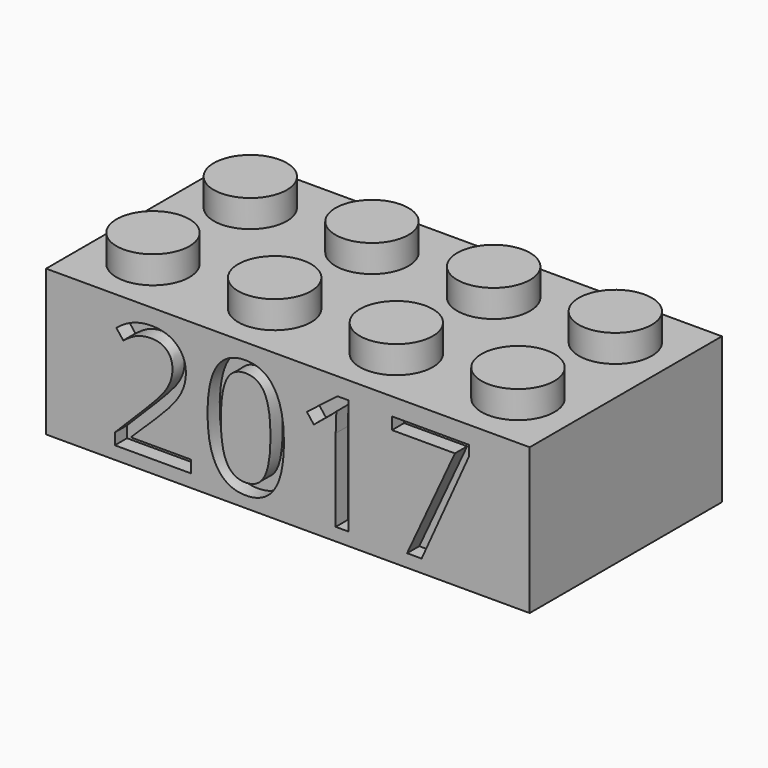
from build123d import *

# Parameters (mm, degrees)
F0_W          = 31.8
F0_H          = 15.8
F1_DEPTH      = 9.6
F2_W          = 29.4
F2_H          = 13.4
F3_DEPTH      = 8.4
F4_R          = 2.4
F5_DEPTH      = 1.8
F6_W          = 29.4
F6_H          = 13.4
F6_R          = 1.3
F7_DEPTH      = 1
F8_R          = 3.255
F9_DEPTH      = 7.4
F10_R         = 2.4
F11_DEPTH     = 7.4
F12_W         = 0.8
F12_H         = 13.4
F13_DEPTH     = 6.4
F15_DEPTH     = 6.4
F16_W         = 0.6
F16_H         = 0.3
F17_DEPTH     = 7.4
F18_W         = 0.3
F18_H         = 0.6
F19_DEPTH     = 7.4
F20_TEXT_SIZE = 9.802063729
F21_DEPTH     = 1
F22_TEXT_SIZE = 10.6435608972
F23_DEPTH     = 1


# Not quite as in the source:
# - Text() gives the source's letters only with a copy of the font that has no kerning and outlines rounded to 1/6400 em; it was checked with that copy


with BuildPart() as f1:
    # F0 (on Top) → F1 (new body)
    with BuildSketch(Plane.XY):
        Rectangle(F0_W, F0_H)
    extrude(amount=F1_DEPTH)

    # F2 (on Top) → F3 (cut)
    with BuildSketch(Plane.XY):
        Rectangle(F2_W, F2_H)
    extrude(amount=F3_DEPTH, mode=Mode.SUBTRACT)

    # F4 (on face) → F5 (join)
    with BuildSketch(Plane.XY.offset(9.6)):
        with Locations((-11.95, 3.95)):
            Circle(F4_R)
        with Locations((-11.95, -4.05)):
            Circle(F4_R)
        with Locations((-3.95, -4.05)):
            Circle(F4_R)
        with Locations((4.05, 3.95)):
            Circle(F4_R)
        with Locations((-3.95, 3.95)):
            Circle(F4_R)
        with Locations((4.05, -4.05)):
            Circle(F4_R)
        with Locations((12.05, -4.05)):
            Circle(F4_R)
        with Locations((12.05, 3.95)):
            Circle(F4_R)
    extrude(amount=F5_DEPTH)

    # F6 (on face) → F7 (join)
    with BuildSketch(Plane(origin=(0, 0, 8.4), x_dir=(1, 0, 0), z_dir=(0, 0, -1))):
        Rectangle(F6_W, F6_H)
        with Locations((-11.95, -4.05)):
            Circle(F6_R, mode=Mode.SUBTRACT)
        with Locations((-3.95, -4.05)):
            Circle(F6_R, mode=Mode.SUBTRACT)
        with Locations((4.05, -4.05)):
            Circle(F6_R, mode=Mode.SUBTRACT)
        with Locations((12.05, -4.05)):
            Circle(F6_R, mode=Mode.SUBTRACT)
        with Locations((-11.95, 3.95)):
            Circle(F6_R, mode=Mode.SUBTRACT)
        with Locations((-3.95, 3.95)):
            Circle(F6_R, mode=Mode.SUBTRACT)
        with Locations((4.05, 3.95)):
            Circle(F6_R, mode=Mode.SUBTRACT)
        with Locations((12.05, 3.95)):
            Circle(F6_R, mode=Mode.SUBTRACT)
    extrude(amount=F7_DEPTH)

    # F8 (on face) → F9 (join)
    with BuildSketch(Plane(origin=(0, 0, 7.4), x_dir=(1, 0, 0), z_dir=(0, 0, -1))):
        with Locations((7.945, 0)):
            Circle(F8_R)
        with Locations((-0.055, 0)):
            Circle(F8_R)
        with Locations((-8.055, 0)):
            Circle(F8_R)
    extrude(amount=F9_DEPTH)

    # F10 (on face) → F11 (cut)
    with BuildSketch(Plane(origin=(0, 0, 0), x_dir=(1, 0, 0), z_dir=(0, 0, -1))):
        with Locations((-8.055, 0)):
            Circle(F10_R)
        with Locations((-0.055, 0)):
            Circle(F10_R)
        with Locations((7.945, 0)):
            Circle(F10_R)
    extrude(amount=-F11_DEPTH, mode=Mode.SUBTRACT)

    # F12 (on face) → F13 (join)
    with BuildSketch(Plane(origin=(0, 0, 7.4), x_dir=(1, 0, 0), z_dir=(0, 0, -1))):
        Rectangle(F12_W, F12_H)
    extrude(amount=F13_DEPTH)

    # F14 (on face) → F15 (cut)
    with BuildSketch(Plane(origin=(0, 0, 1), x_dir=(1, 0, 0), z_dir=(0, 0, -1))):
        with BuildLine():
            Line((-0.4, 2.3750736831), (-0.4, -2.3750736831))
            ThreePointArc((-0.4, -2.3750736831), (0.0007806115, -2.3993516881), (0.4, -2.3564751219))
            Line((0.4, -2.3564751219), (0.4, 2.3564751219))
            ThreePointArc((0.4, 2.3564751219), (0.0007806115, 2.3993516881), (-0.4, 2.3750736831))
        make_face()
    extrude(amount=-F15_DEPTH, mode=Mode.SUBTRACT)

    # F16 (on face) → F17 (join, through all)
    with BuildSketch(Plane(origin=(0, 0, 0), x_dir=(1, 0, 0), z_dir=(0, 0, -1))):
        with Locations((-11.95, 6.55)):
            Rectangle(F16_W, F16_H)
        with Locations((-11.95, -6.55)):
            Rectangle(F16_W, F16_H)
        with Locations((-3.95, 6.55)):
            Rectangle(F16_W, F16_H)
        with Locations((-3.95, -6.55)):
            Rectangle(F16_W, F16_H)
        with Locations((4.05, 6.55)):
            Rectangle(F16_W, F16_H)
        with Locations((4.05, -6.55)):
            Rectangle(F16_W, F16_H)
        with Locations((12.05, 6.55)):
            Rectangle(F16_W, F16_H)
        with Locations((12.05, -6.55)):
            Rectangle(F16_W, F16_H)
    extrude(amount=-F17_DEPTH)

    # F18 (on face) → F19 (join, through all)
    with BuildSketch(Plane(origin=(0, 0, 0), x_dir=(1, 0, 0), z_dir=(0, 0, -1))):
        with Locations((-14.55, 4.05)):
            Rectangle(F18_W, F18_H)
        with Locations((-14.55, -3.95)):
            Rectangle(F18_W, F18_H)
        with Locations((14.55, 4.05)):
            Rectangle(F18_W, F18_H)
        with Locations((14.55, -3.95)):
            Rectangle(F18_W, F18_H)
    extrude(amount=-F19_DEPTH)

    # F20 (on face) → F21 (cut)
    with BuildSketch(Plane(origin=(0, 7.9, 0), x_dir=(-1, 0, 0), z_dir=(0, 1, 0))):
        with Locations((-11.8, 1.3417988588)):
            Text('Dane', F20_TEXT_SIZE, font='Open Sans', text_align=(TextAlign.LEFT, TextAlign.BOTTOM))
    extrude(amount=-F21_DEPTH, mode=Mode.SUBTRACT)

    # F22 (on face) → F23 (cut)
    with BuildSketch(Plane.XZ.offset(7.9)):
        with Locations((-11.9, 0.8446492609)):
            Text('2017', F22_TEXT_SIZE, font='Open Sans', text_align=(TextAlign.LEFT, TextAlign.BOTTOM))
    extrude(amount=-F23_DEPTH, mode=Mode.SUBTRACT)


solid = f1.part
